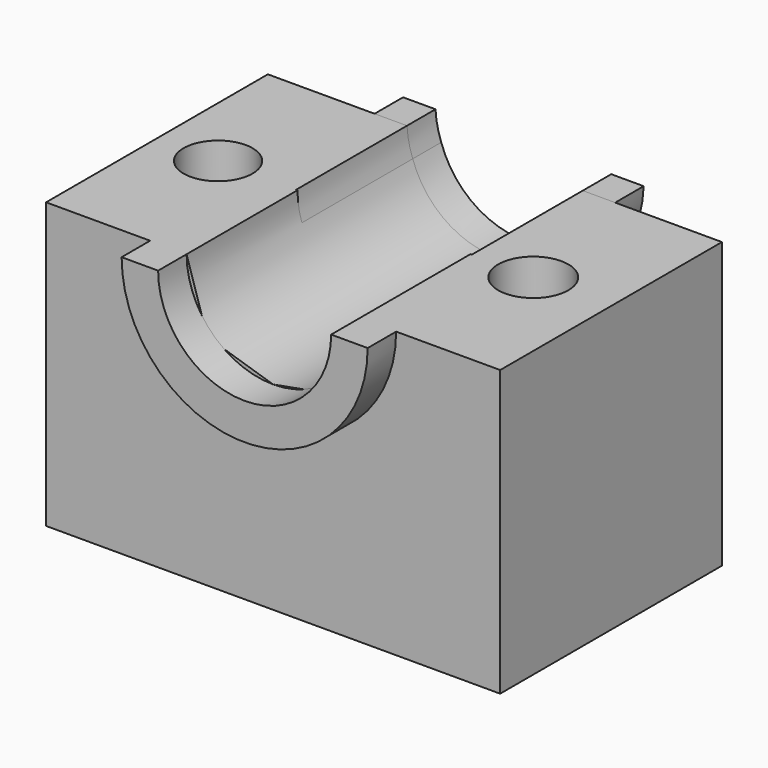
from build123d import *

# Parameters (mm, degrees)
F0_W     = 80.9574872255
F0_H     = 49.4184233248
F0_R     = 6.1446499531
F0_R_2   = 6.2581528025
F1_DEPTH = 50.8
F3_DEPTH = 24.7092116624
F5_DEPTH = 49.4194233248
F7_DEPTH = 6.35
F9_DEPTH = 6.35


# Not quite as in the source:
# - ends of sketch curves that miss each other by under 0.0002 mm in the source are joined


with BuildPart() as f1:
    # F0 (on Top) → F1 (new body)
    with BuildSketch(Plane.XY):
        Rectangle(F0_W, F0_H)
        with Locations((-29.5835565776, 0)):
            Circle(F0_R, mode=Mode.SUBTRACT)
        with Locations((26.6144089401, 0)):
            Circle(F0_R_2, mode=Mode.SUBTRACT)
    extrude(amount=F1_DEPTH)

    # F2 (on Front) → F3 (cut, through all)
    with BuildSketch(Plane.XZ):
        with BuildLine():
            Line((15.6650725744, 50.8), (-15.6650725744, 50.8))
            ThreePointArc((-15.6650725744, 50.8), (0, 35.8885951003), (15.6650725744, 50.8))
        make_face()
    extrude(amount=-F3_DEPTH, mode=Mode.SUBTRACT)

    # F4 (on face) → F5 (cut, through all)
    with BuildSketch(Plane.XZ.offset(24.7092116624)):
        with BuildLine():
            Line((15.4236163944, 50.8), (-15.4236244361, 50.8))
            ThreePointArc((-15.4236244361, 50.8), (0, 35.3763755639), (15.4236163944, 50.8))
        make_face()
    extrude(amount=-F5_DEPTH, mode=Mode.SUBTRACT)

    # F8 (on face) → F9 (join)
    with BuildSketch(Plane.XZ.offset(24.7092116624)):
        with BuildLine():
            ThreePointArc((15.4236244361, 50.8), (0, 35.3763755639), (-15.4236244361, 50.8))
            Line((-15.4236244361, 50.8), (-21.9304505736, 50.8))
            ThreePointArc((-21.9304505736, 50.8), (0, 28.8695494264), (21.9304505736, 50.8))
            Line((21.9304505736, 50.8), (15.4236244361, 50.8))
        make_face()
    extrude(amount=F9_DEPTH)


with BuildPart() as f7:
    # F6 (on face) → F7 (new body)
    with BuildSketch(Plane(origin=(0, 24.7092116624, 0), x_dir=(-1, 0, 0), z_dir=(0, 1, 0))):
        with BuildLine():
            ThreePointArc((-14.638826209, 45.9427625882), (-15.3453497577, 48.3305192967), (-15.6650725744, 50.8))
            Line((-15.6650725744, 50.8), (-21.4484650642, 50.8))
            ThreePointArc((-21.4484650642, 50.8), (0, 30.1103343441), (21.4484650642, 50.8))
            Line((21.4484650642, 50.8), (15.6650725744, 50.8))
            ThreePointArc((15.6650725744, 50.8), (15.3453666282, 48.330599146), (14.638884799, 45.9429149343))
            ThreePointArc((14.638884799, 45.9429149343), (8.42774e-05, 35.3763755642), (-14.638826209, 45.9427625882))
        make_face()
    extrude(amount=F7_DEPTH)


solid = Compound([f1.part, f7.part])
